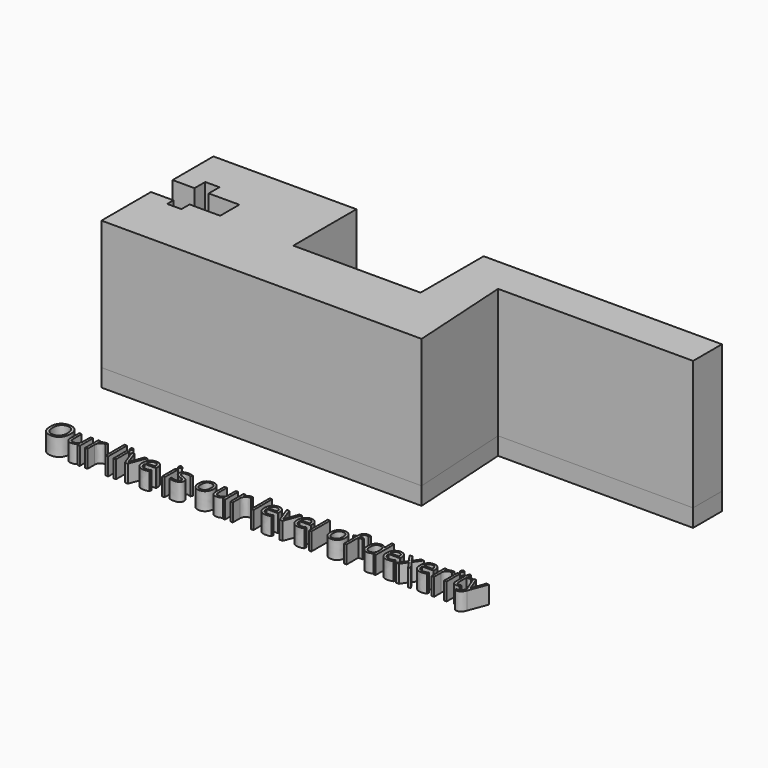
from build123d import *

# Parameters (mm, degrees)
F1_DEPTH     = 3
F2_DEPTH     = 25
F0_TEXT_SIZE = 5.2506673253
F3_DEPTH     = 3


# Not quite as in the source:
# - Text() gives the source's letters only with a copy of the font that has no kerning and outlines rounded to 1/6400 em; it was checked with that copy


with BuildPart() as f1:
    # F0 (on Top) → F1 (new body)
    with BuildSketch(Plane.XY):
        Polygon((-113.6067956686, 48.6474893987), (-137.9160583019, 48.6474893987), (-137.9022598267, 39.9532690644), (-134.1710686684, 39.9532690644), (-134.1710686684, 42.2289855778), (-131.7556649446, 42.2289855778), (-131.7556649446, 39.9532690644), (-126.5574246645, 39.9532690644), (-126.5574246645, 35.8854793012), (-131.7556649446, 35.8854793012), (-131.7556649446, 34.153111279), (-134.1710686684, 34.153111279), (-134.1710686684, 35.4785844684), (-137.9967480898, 35.4785844684), (-137.9967480898, 24.9479042711), (-83.5496162081, 24.9479042711), (-84.6162810922, 42.5216071308), (-51.4525622129, 42.5216071308), (-51.4525622129, 48.6474893987), (-91.9674262404, 48.6474893987), (-91.9674262404, 35.2368690073), (-113.6067956686, 35.2368690073), align=None)
    extrude(amount=F1_DEPTH)


with BuildPart() as f2:
    # F0 (on Top) → F2 (new body)
    with BuildSketch(Plane.XY):
        Polygon((-113.6067956686, 48.6474893987), (-137.9160583019, 48.6474893987), (-137.9022598267, 39.9532690644), (-134.1710686684, 39.9532690644), (-134.1710686684, 42.2289855778), (-131.7556649446, 42.2289855778), (-131.7556649446, 39.9532690644), (-126.5574246645, 39.9532690644), (-126.5574246645, 35.8854793012), (-131.7556649446, 35.8854793012), (-131.7556649446, 34.153111279), (-134.1710686684, 34.153111279), (-134.1710686684, 35.4785844684), (-137.9967480898, 35.4785844684), (-137.9967480898, 24.9479042711), (-83.5496162081, 24.9479042711), (-84.6162810922, 42.5216071308), (-51.4525622129, 42.5216071308), (-51.4525622129, 48.6474893987), (-91.9674262404, 48.6474893987), (-91.9674262404, 35.2368690073), (-113.6067956686, 35.2368690073), align=None)
    extrude(amount=F2_DEPTH)


with BuildPart() as f3:
    # F0 (on Top) → F3 (new body)
    with BuildSketch(Plane.XY):
        Polygon((-113.6067956686, 48.6474893987), (-137.9160583019, 48.6474893987), (-137.9022598267, 39.9532690644), (-134.1710686684, 39.9532690644), (-134.1710686684, 42.2289855778), (-131.7556649446, 42.2289855778), (-131.7556649446, 39.9532690644), (-126.5574246645, 39.9532690644), (-126.5574246645, 35.8854793012), (-131.7556649446, 35.8854793012), (-131.7556649446, 34.153111279), (-134.1710686684, 34.153111279), (-134.1710686684, 35.4785844684), (-137.9967480898, 35.4785844684), (-137.9967480898, 24.9479042711), (-83.5496162081, 24.9479042711), (-84.6162810922, 42.5216071308), (-51.4525622129, 42.5216071308), (-51.4525622129, 48.6474893987), (-91.9674262404, 48.6474893987), (-91.9674262404, 35.2368690073), (-113.6067956686, 35.2368690073), align=None)
        with Locations((-133.0346018076, 5.5614458397)):
            Text('Our live is our level of dexerity', F0_TEXT_SIZE, font='Open Sans', text_align=(TextAlign.LEFT, TextAlign.BOTTOM))
    extrude(amount=F3_DEPTH)


solid = Compound([f1.part, f2.part, f3.part])
